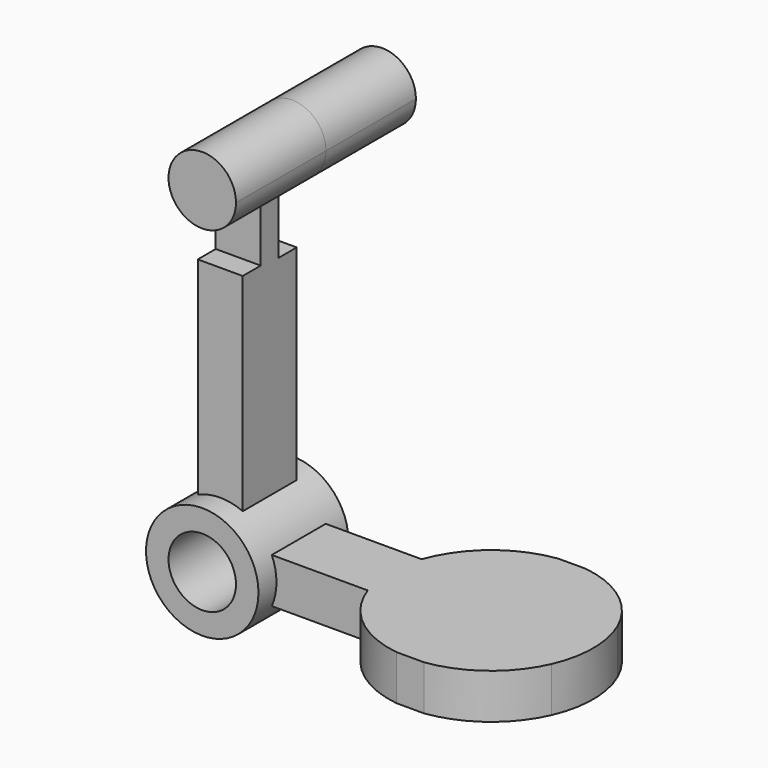
from build123d import *
from build123d import SkipClean  # not in build123d's __all__

# Parameters (mm, degrees)
F0_R           = 6.35
F0_R_2         = 3.81
F1_DEPTH       = 12.7
F4_DEPTH       = 38.1
F5_DEPTH       = 25.4
F5_DEPTH_BACK  = 25.4
F6_W           = 13.8230553448
F6_H           = 5.08
F7_DEPTH       = 7.62
F7_DEPTH_BACK  = 15.24
F8_DEPTH       = 7.62
F9_DEPTH       = 7.62
F11_DEPTH      = 25.4
F12_DEPTH      = 5.08
F14_DEPTH      = 38.1
F15_DEPTH      = 25.4
F16_W          = 2.54
F16_H          = 9.144
F17_DEPTH      = 2.54
F18_W          = 2.54
F18_H          = 8.89
F19_DEPTH      = 2.54
F21_DEPTH      = 12.7
F21_DEPTH_BACK = 12.7


with BuildPart() as f1:
    # F0 (on Front) → F1 (new body)
    with BuildSketch(Plane.XZ):
        Circle(F0_R)
        Circle(F0_R_2, mode=Mode.SUBTRACT)
    extrude(amount=F1_DEPTH)

    # F3 (on Right) → F4 (join)
    with BuildSketch(Plane.YZ):
        Polygon((-2.54, -2.54), (-2.54, 0), (-2.54, 2.54), (-10.16, 2.54), (-10.16, 0), (-10.16, -2.54), align=None)
    extrude(amount=F4_DEPTH)

    # F0 (on Front) → F5 (cut, two sides)
    with BuildSketch(Plane.XZ) as f5_sk:
        Circle(F0_R_2)
    extrude(amount=F5_DEPTH, mode=Mode.SUBTRACT)
    extrude(f5_sk.sketch, amount=-F5_DEPTH_BACK, mode=Mode.SUBTRACT)

    # F6 (on face) → F7 (join, two sides)
    with BuildSketch(Plane.XZ.offset(10.16)) as f7_sk:
        with Locations((31.1884723276, 0)):
            Rectangle(F6_W, F6_H)
    extrude(amount=F7_DEPTH)
    extrude(f7_sk.sketch, amount=-F7_DEPTH_BACK)

    # F8 (add): a face of the model
    f8_faces = [f1.faces().sort_by_distance(p)[0] for p in [
        (24.2769446552, -13.97, 0),
    ]]
    extrude(f8_faces, amount=F8_DEPTH)

    # F9 (add): a face of the model
    f9_faces = [f1.faces().sort_by_distance(p)[0] for p in [
        (24.2769446552, 1.27, 0),
    ]]
    extrude(f9_faces, amount=F9_DEPTH)

    # F10 (on face) → F11 (cut)
    with BuildSketch(Plane.XY.offset(2.54)):
        with BuildLine():
            ThreePointArc((25.9835010893, -17.78), (20.2469210754, -15.2836758241), (16.6569446552, -10.16))
            Line((16.6569446552, -10.16), (16.6569446552, -17.78))
            Line((16.6569446552, -17.78), (25.9835010893, -17.78))
        make_face()
        with BuildLine():
            Line((16.6569446552, 5.08), (16.6569446552, -2.54))
            ThreePointArc((16.6569446552, -2.54), (20.2469210754, 2.5836758241), (25.9835010893, 5.08))
            Line((25.9835010893, 5.08), (16.6569446552, 5.08))
        make_face()
        with BuildLine():
            Line((38.1, 5.08), (29.1083570088, 5.08))
            ThreePointArc((29.1083570088, 5.08), (34.4861831348, 2.8651480918), (38.1, -1.6919244863))
            Line((38.1, -1.6919244863), (38.1, 5.08))
        make_face()
        with BuildLine():
            Line((38.1, -17.78), (38.1, -11.0080755137))
            ThreePointArc((38.1, -11.0080755137), (34.4861831348, -15.5651480918), (29.1083570088, -17.78))
            Line((29.1083570088, -17.78), (38.1, -17.78))
        make_face()
    extrude(amount=-F11_DEPTH, mode=Mode.SUBTRACT)

    # F10 (on face) → F12 (join)
    with BuildSketch(Plane.XY.offset(2.54)):
        with BuildLine():
            ThreePointArc((38.1, -11.0080755137), (39.0822231303, -6.35), (38.1, -1.6919244863))
            Line((38.1, -1.6919244863), (38.1, -11.0080755137))
        make_face()
    with SkipClean():  # cleaning this boolean's faces spoils the solid; the shape is the same uncleaned
        extrude(amount=-F12_DEPTH)

    # F13 (on Top) → F14 (join)
    with BuildSketch(Plane.XY):
        Polygon((2.54, -2.54), (0, -2.54), (-2.54, -2.54), (-2.54, -10.16), (0, -10.16), (2.54, -10.16), align=None)
    extrude(amount=F14_DEPTH)

    # F0 (on Front) → F15 (cut)
    with BuildSketch(Plane.XZ):
        Circle(F0_R_2)
    extrude(amount=F15_DEPTH, mode=Mode.SUBTRACT)

    # F16 (on face) → F17 (cut)
    with BuildSketch(Plane(origin=(0, -2.54, 0), x_dir=(-1, 0, 0), z_dir=(0, 1, 0))):
        with Locations((-1.27, 33.528)):
            Rectangle(F16_W, F16_H)
        with Locations((1.27, 33.528)):
            Rectangle(F16_W, F16_H)
    extrude(amount=-F17_DEPTH, mode=Mode.SUBTRACT)

    # F18 (on face) → F19 (cut)
    with BuildSketch(Plane.XZ.offset(10.16)):
        with Locations((-1.27, 33.655)):
            Rectangle(F18_W, F18_H)
        with Locations((1.27, 33.655)):
            Rectangle(F18_W, F18_H)
    extrude(amount=-F19_DEPTH, mode=Mode.SUBTRACT)

    # F20 (on Front) → F21 (join, two sides)
    with BuildSketch(Plane.XZ) as f21_sk:
        with BuildLine():
            ThreePointArc((0, 34.1351066256), (2.6940768363, 35.2510297892), (3.81, 37.9451066256))
            ThreePointArc((3.81, 37.9451066256), (-2.6940768363, 40.6391834619), (0, 34.1351066256))
        make_face()
    extrude(amount=F21_DEPTH)
    extrude(f21_sk.sketch, amount=-F21_DEPTH_BACK)


solid = f1.part
